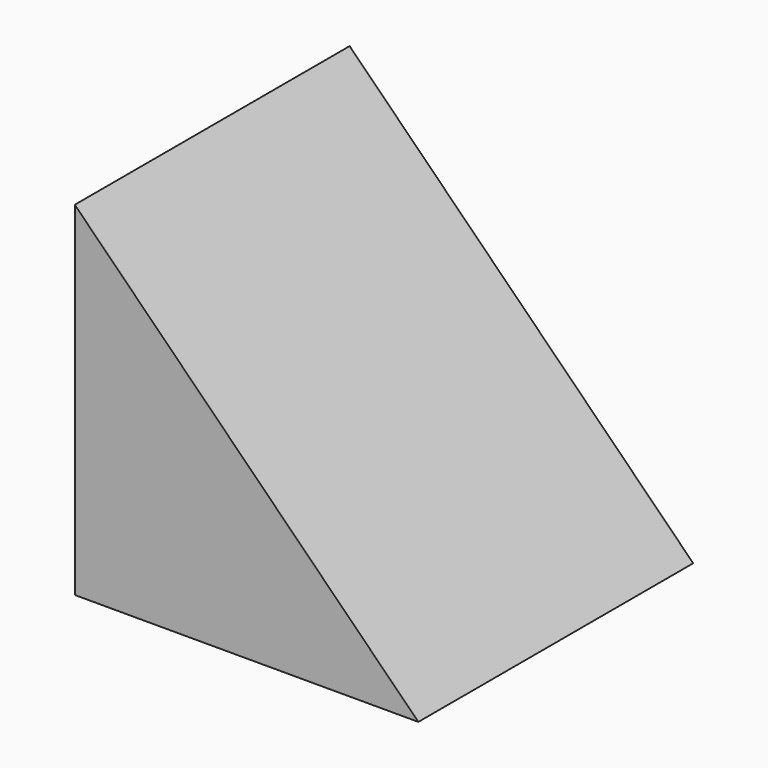
from build123d import *

# Parameters (mm, degrees)
F0_W          = 40
F0_H          = 40
F1_DEPTH      = 20
F1_DEPTH_BACK = 20
F2_SIZE       = 39.99999


# Not quite as in the source:
# - a fillet or chamfer is up to 0.001 mm smaller than in the source, because OpenCascade refuses the exact size


with BuildPart() as f1:
    # F0 (on Top) → F1 (new body, two sides)
    with BuildSketch(Plane.XY) as f1_sk:
        Rectangle(F0_W, F0_H)
    extrude(amount=F1_DEPTH)
    extrude(f1_sk.sketch, amount=-F1_DEPTH_BACK)

    # F2 (size 40 in the source; OpenCascade refuses exactly that, so slightly less here)
    f2_edges = [f1.edges().sort_by_distance(p)[0] for p in [
        (20, 0, 20),
    ]]
    chamfer(f2_edges, length=F2_SIZE)


solid = f1.part
